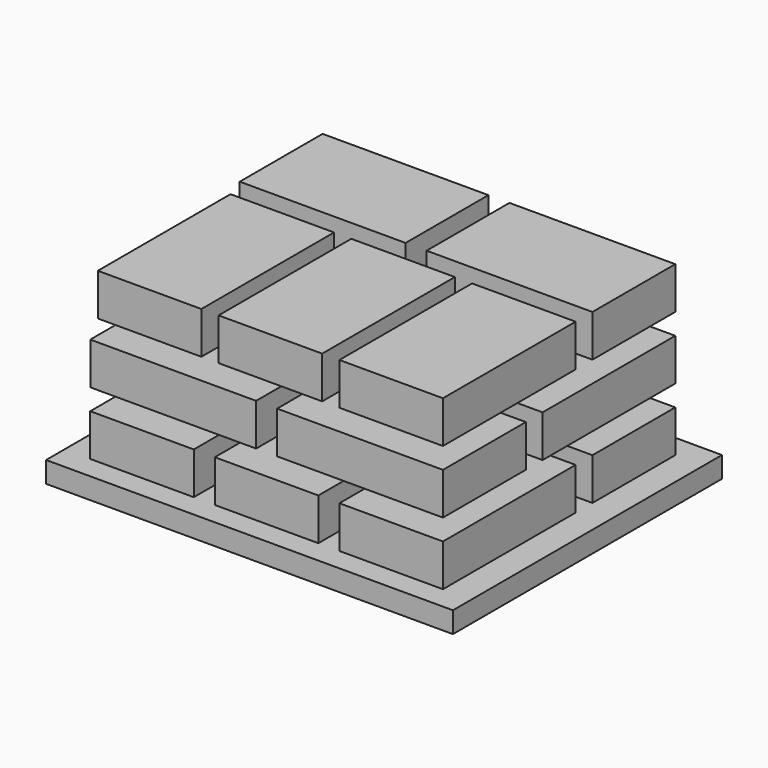
from build123d import *

# Parameters (mm, degrees)
F0_W     = 20.0432797
F0_H     = 12.5155309215
F1_DEPTH = 5.08
F0_W_2   = 12.5155309215
F0_H_2   = 20.0432797
F2_W     = 49.1681545973
F2_H     = 2.54
F3_DEPTH = 20.32
F5_W     = 12.5155309215
F5_H     = 20.0432797
F6_DEPTH = 5.08
F5_W_2   = 20.0432797
F5_H_2   = 12.5155309215
F8_W     = 20.0432797
F8_H     = 12.5155309215
F9_DEPTH = 5.08
F8_W_2   = 12.5155309215
F8_H_2   = 20.0432797


with BuildPart() as f1:
    # F0 (on Top) → F1 (new body)
    with BuildSketch(Plane.XY):
        with Locations((11.29163985, 11.2916406392)):
            Rectangle(F0_W, F0_H)
    extrude(amount=F1_DEPTH)


with BuildPart() as f1b:
    # F0 (on Top) → F1, piece 2 (new body)
    with BuildSketch(Plane.XY):
        with Locations((15.0555253608, -7.5277646715)):
            Rectangle(F0_W_2, F0_H_2)
    extrude(amount=F1_DEPTH)


with BuildPart() as f1c:
    # F0 (on Top) → F1, piece 3 (new body)
    with BuildSketch(Plane.XY):
        with Locations((-5.5608e-06, -7.5277646715)):
            Rectangle(F0_W_2, F0_H_2)
    extrude(amount=F1_DEPTH)


with BuildPart() as f1d:
    # F0 (on Top) → F1, piece 4 (new body)
    with BuildSketch(Plane.XY):
        with Locations((-15.0555364823, -7.5277646715)):
            Rectangle(F0_W_2, F0_H_2)
    extrude(amount=F1_DEPTH)


with BuildPart() as f1e:
    # F0 (on Top) → F1, piece 5 (new body)
    with BuildSketch(Plane.XY):
        with Locations((-11.29163985, 11.2916406392)):
            Rectangle(F0_W, F0_H)
    extrude(amount=F1_DEPTH)


with BuildPart() as f3:
    # F2 (on Front) → F3 (new body, symmetric)
    with BuildSketch(Plane.XZ):
        with Locations((0.1489929855, -1.27)):
            Rectangle(F2_W, F2_H)
    extrude(amount=F3_DEPTH, both=True)


with BuildPart() as f6:
    # F5 (on offset) → F6 (new body)
    with BuildSketch(Plane.XY.offset(7.62)):
        with Locations((5.5608e-06, 7.52776625)):
            Rectangle(F5_W, F5_H)
    extrude(amount=F6_DEPTH)


with BuildPart() as f6b:
    # F5 (on offset) → F6, piece 2 (new body)
    with BuildSketch(Plane.XY.offset(7.62)):
        with Locations((15.0555253608, 7.52776625)):
            Rectangle(F5_W, F5_H)
    extrude(amount=F6_DEPTH)


with BuildPart() as f6c:
    # F5 (on offset) → F6, piece 3 (new body)
    with BuildSketch(Plane.XY.offset(7.62)):
        with Locations((11.2916509715, -11.2916390608)):
            Rectangle(F5_W_2, F5_H_2)
    extrude(amount=F6_DEPTH)


with BuildPart() as f6d:
    # F5 (on offset) → F6, piece 4 (new body)
    with BuildSketch(Plane.XY.offset(7.62)):
        with Locations((-11.2916287285, -11.2916390608)):
            Rectangle(F5_W_2, F5_H_2)
    extrude(amount=F6_DEPTH)


with BuildPart() as f6e:
    # F5 (on offset) → F6, piece 5 (new body)
    with BuildSketch(Plane.XY.offset(7.62)):
        with Locations((-15.0555142392, 7.52776625)):
            Rectangle(F5_W, F5_H)
    extrude(amount=F6_DEPTH)


with BuildPart() as f9:
    # F8 (on offset) → F9 (new body)
    with BuildSketch(Plane.XY.offset(15.24)):
        with Locations((-11.29163985, 11.2916406392)):
            Rectangle(F8_W, F8_H)
    extrude(amount=F9_DEPTH)


with BuildPart() as f9b:
    # F8 (on offset) → F9, piece 2 (new body)
    with BuildSketch(Plane.XY.offset(15.24)):
        with Locations((11.2916509715, 11.2916406392)):
            Rectangle(F8_W, F8_H)
    extrude(amount=F9_DEPTH)


with BuildPart() as f9c:
    # F8 (on offset) → F9, piece 3 (new body)
    with BuildSketch(Plane.XY.offset(15.24)):
        with Locations((15.0555253608, -7.5277646715)):
            Rectangle(F8_W_2, F8_H_2)
    extrude(amount=F9_DEPTH)


with BuildPart() as f9d:
    # F8 (on offset) → F9, piece 4 (new body)
    with BuildSketch(Plane.XY.offset(15.24)):
        with Locations((0.4578256088, -7.5277646715)):
            Rectangle(F8_W_2, F8_H_2)
    extrude(amount=F9_DEPTH)


with BuildPart() as f9e:
    # F8 (on offset) → F9, piece 5 (new body)
    with BuildSketch(Plane.XY.offset(15.24)):
        with Locations((-14.1398741431, -7.5277646715)):
            Rectangle(F8_W_2, F8_H_2)
    extrude(amount=F9_DEPTH)


solid = Compound([f1.part, f1b.part, f1c.part, f1d.part, f1e.part, f3.part, f6.part, f6b.part, f6c.part, f6d.part, f6e.part, f9.part, f9b.part, f9c.part, f9d.part, f9e.part])
